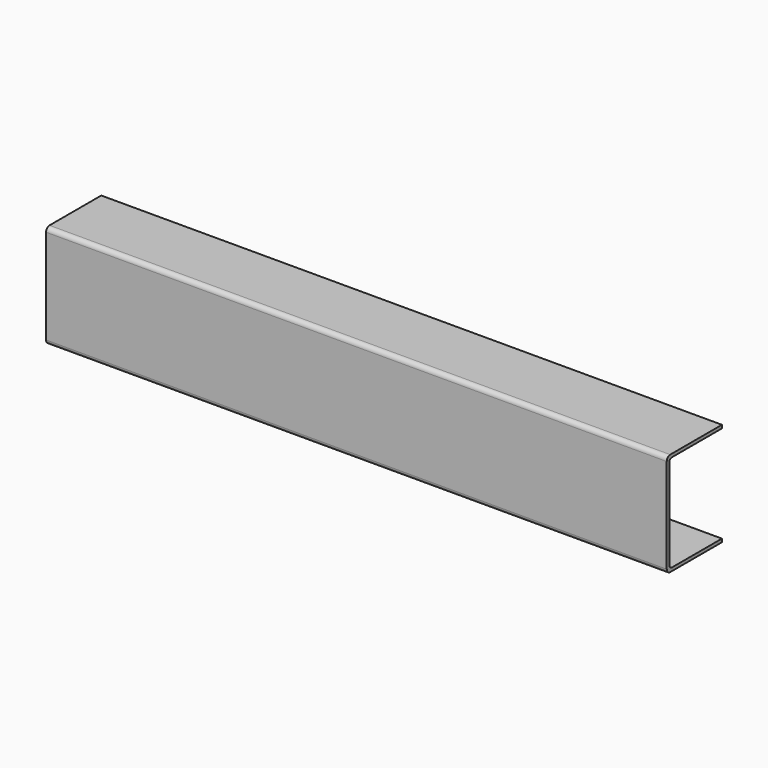
from build123d import *

# Parameters (mm, degrees)
F1_DEPTH      = 457.2
F1_DEPTH_BACK = 457.2


with BuildPart() as f1:
    # F0 (on Right) → F1 (new body, two sides)
    with BuildSketch(Plane.YZ) as f1_sk:
        with BuildLine():
            Line((101.6, 71.4375), (101.6, 76.2))
            Line((101.6, 76.2), (6.35, 76.2))
            ThreePointArc((6.35, 76.2), (1.8598719395, 74.3401280605), (0, 69.85))
            Line((0, 69.85), (0, 0))
            Line((0, 0), (0, -69.85))
            ThreePointArc((0, -69.85), (1.8598719395, -74.3401280605), (6.35, -76.2))
            Line((6.35, -76.2), (101.6, -76.2))
            Line((101.6, -76.2), (101.6, -71.4375))
            Line((101.6, -71.4375), (9.525, -71.4375))
            ThreePointArc((9.525, -71.4375), (6.1574039546, -70.0425960454), (4.7625, -66.675))
            Line((4.7625, -66.675), (4.7625, 0))
            Line((4.7625, 0), (4.7625, 66.675))
            ThreePointArc((4.7625, 66.675), (6.1574039546, 70.0425960454), (9.525, 71.4375))
            Line((9.525, 71.4375), (101.6, 71.4375))
        make_face()
    extrude(amount=-F1_DEPTH)
    extrude(f1_sk.sketch, amount=F1_DEPTH_BACK)


solid = f1.part
